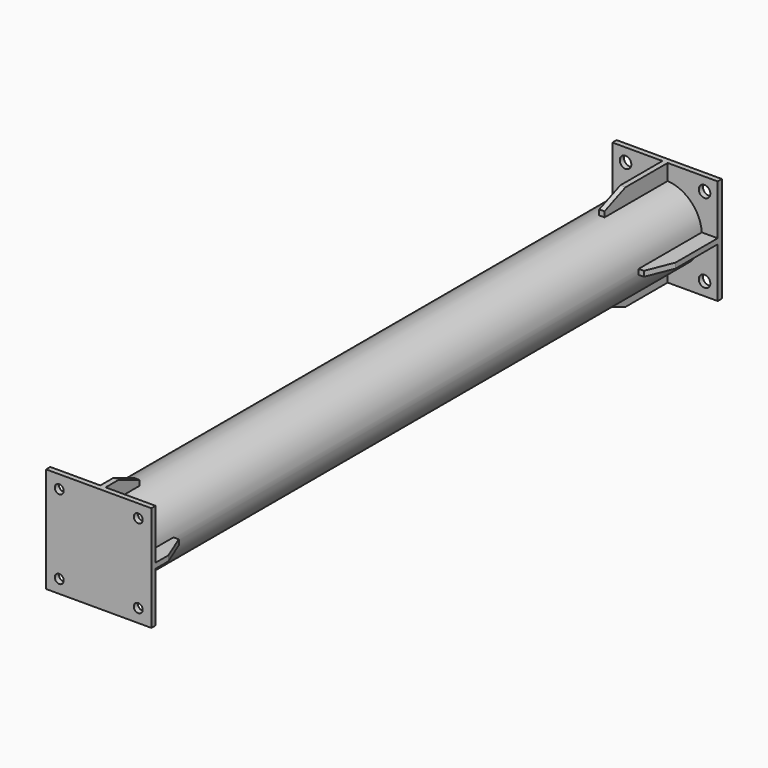
from build123d import *

# Parameters (mm, degrees)
F0_R          = 70
F0_R_2        = 65
F1_DEPTH      = 1334
F2_W          = 200
F2_H          = 200
F2_R          = 11
F3_DEPTH      = 10
F4_W          = 30.1787997812
F4_H          = 10
F4_W_2        = 10
F4_H_2        = 30.1787997812
F5_DEPTH      = 150
F6_T1_DEPTH   = 269.311363913
F6_T3_DEPTH   = 269.311363913
F6_T8_DEPTH   = 269.311363913
F6_S9_R       = 70
F6_T10_DEPTH  = 139
F8_W          = 200
F8_H          = 200
F8_R          = 8.5
F9_DEPTH      = 10
F10_W         = 10
F10_H         = 30.1787997812
F10_W_2       = 30.1787997812
F10_H_2       = 10
F11_DEPTH     = 80
F12_T1_DEPTH  = 269.311363913
F12_T3_DEPTH  = 269.311363913
F12_T8_DEPTH  = 269.311363913
F12_S9_R      = 70
F12_T10_DEPTH = 139
F12_T14_DEPTH = 269.311363913
F12_S15_R     = 70
F12_T16_DEPTH = 139


# Not quite as in the source:
# - a fillet or chamfer that OpenCascade refuses, or shapes differently, is made with other operations: its cross-section is extruded or revolved along the edge and cut away or added


with BuildPart() as f1:
    # F0 (on Front) → F1 (new body)
    with BuildSketch(Plane.XZ):
        Circle(F0_R)
        Circle(F0_R_2, mode=Mode.SUBTRACT)
    extrude(amount=F1_DEPTH)

    # F2 (on Front) → F3 (join)
    with BuildSketch(Plane.XZ):
        Rectangle(F2_W, F2_H)
        with Locations((-75, -75)):
            Circle(F2_R, mode=Mode.SUBTRACT)
        with Locations((75, -75)):
            Circle(F2_R, mode=Mode.SUBTRACT)
        with Locations((-75, 75)):
            Circle(F2_R, mode=Mode.SUBTRACT)
        with Locations((75, 75)):
            Circle(F2_R, mode=Mode.SUBTRACT)
    extrude(amount=-F3_DEPTH)

    # F4 (on Front) → F5 (join)
    with BuildSketch(Plane.XZ):
        with Locations((-84.9106001094, 0)):
            Rectangle(F4_W, F4_H)
        with Locations((0, 84.9106001094)):
            Rectangle(F4_W_2, F4_H_2)
        with Locations((84.9106001094, 0)):
            Rectangle(F4_W, F4_H)
        with Locations((0, -84.9106001094)):
            Rectangle(F4_W_2, F4_H_2)
    extrude(amount=F5_DEPTH)

    # F6: chamfer of 50 x 20 on 4 edges, made by hand

    # F6_s2 → F6_t1 (cut)
    with BuildSketch(Plane.YZ.offset(-134.6556819565)):
        Polygon((-100, 100), (-150, 80), (-150, 100), align=None)
        Polygon((-100, -100), (-150, -80), (-150, -100), align=None)
    extrude(amount=F6_T1_DEPTH, mode=Mode.SUBTRACT)

    # F6_s4 → F6_t3 (cut)
    with BuildSketch(Plane.XY.offset(-134.6556819565)):
        Polygon((100, -100), (80, -150), (100, -150), align=None)
    extrude(amount=F6_T3_DEPTH, mode=Mode.SUBTRACT)


with BuildPart() as f6_tool6:
    # F6_s7 → F6_t8 (new body)
    with BuildSketch(Plane.XY.offset(134.6556819565)):
        Polygon((-100, -130), (-50, -150), (-100, -150), align=None)
    extrude(amount=-F6_T8_DEPTH)

    # F6_s9 → F6_t10 (cut, symmetric)
    with BuildSketch(Plane.XZ.offset(140)):
        Circle(F6_S9_R)
    extrude(amount=F6_T10_DEPTH, both=True, mode=Mode.SUBTRACT)


with BuildPart() as f1_1:
    add(f1.part)

    # F6_t5: cut F6_tool6
    add(f6_tool6.part, mode=Mode.SUBTRACT)

    # F8 (on offset) → F9 (join)
    with BuildSketch(Plane.XZ.offset(1334)):
        Rectangle(F8_W, F8_H)
        with Locations((-75, -75)):
            Circle(F8_R, mode=Mode.SUBTRACT)
        with Locations((75, -75)):
            Circle(F8_R, mode=Mode.SUBTRACT)
        with Locations((-75, 75)):
            Circle(F8_R, mode=Mode.SUBTRACT)
        with Locations((75, 75)):
            Circle(F8_R, mode=Mode.SUBTRACT)
    extrude(amount=F9_DEPTH)

    # F10 (on face) → F11 (join)
    with BuildSketch(Plane(origin=(0, -1334, 0), x_dir=(-1, 0, 0), z_dir=(0, 1, 0))):
        with Locations((0, 84.9106001094)):
            Rectangle(F10_W, F10_H)
        with Locations((84.9106001094, 0)):
            Rectangle(F10_W_2, F10_H_2)
        with Locations((0, -84.9106001094)):
            Rectangle(F10_W, F10_H)
        with Locations((-84.9106001094, 0)):
            Rectangle(F10_W_2, F10_H_2)
    extrude(amount=F11_DEPTH)

    # F12: chamfer of 20 x 50 on 4 edges, made by hand

    # F12_s2 → F12_t1 (cut)
    with BuildSketch(Plane.YZ.offset(-134.6556819565)):
        Polygon((-1304, 100), (-1254, 80), (-1254, 100), align=None)
    extrude(amount=F12_T1_DEPTH, mode=Mode.SUBTRACT)

    # F12_s4 → F12_t3 (cut)
    with BuildSketch(Plane.XY.offset(-134.6556819565)):
        Polygon((100, -1304), (80, -1254), (100, -1254), align=None)
    extrude(amount=F12_T3_DEPTH, mode=Mode.SUBTRACT)


with BuildPart() as f12_tool6:
    # F12_s7 → F12_t8 (new body)
    with BuildSketch(Plane.XY.offset(-134.6556819565)):
        Polygon((-100, -1274), (-50, -1254), (-100, -1254), align=None)
    extrude(amount=F12_T8_DEPTH)

    # F12_s9 → F12_t10 (cut, symmetric)
    with BuildSketch(Plane.XZ.offset(1264)):
        Circle(F12_S9_R)
    extrude(amount=F12_T10_DEPTH, both=True, mode=Mode.SUBTRACT)


with BuildPart() as f1_2:
    add(f1_1.part)

    # F12_t5: cut F12_tool6
    add(f12_tool6.part, mode=Mode.SUBTRACT)


with BuildPart() as f12_tool12:
    # F12_s13 → F12_t14 (new body)
    with BuildSketch(Plane.YZ.offset(134.6556819565)):
        Polygon((-1274, -100), (-1254, -50), (-1254, -100), align=None)
    extrude(amount=-F12_T14_DEPTH)

    # F12_s15 → F12_t16 (cut, symmetric)
    with BuildSketch(Plane.XZ.offset(1264)):
        Circle(F12_S15_R)
    extrude(amount=F12_T16_DEPTH, both=True, mode=Mode.SUBTRACT)


with BuildPart() as f1_3:
    add(f1_2.part)

    # F12_t11: cut F12_tool12
    add(f12_tool12.part, mode=Mode.SUBTRACT)


solid = f1_3.part
